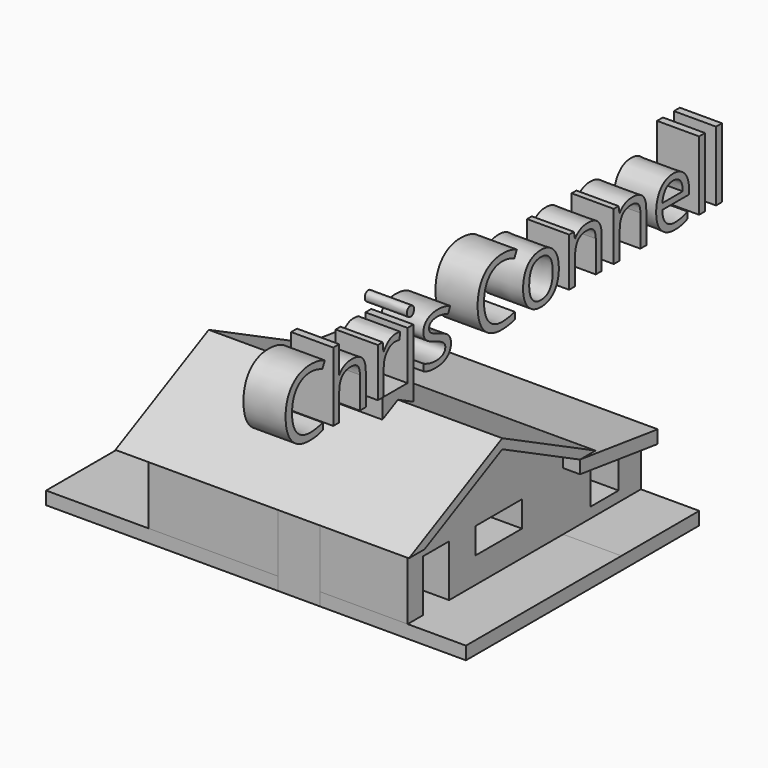
from build123d import *

# Parameters (mm, degrees)
F0_W           = 228.6
F0_H           = 101.6
F0_W_2         = 137.1599945068
F0_H_2         = 137.1599945068
F1_DEPTH       = 508
F0_W_3         = 76.2
F0_H_3         = 177.8
F2_DEPTH       = 530.86
F0_W_4         = 203.2000002861
F0_H_4         = 76.2000002861
F0_W_5         = 101.6
F3_DEPTH       = 736.6
F4_DEPTH       = 909.32
F0_TEXT_SIZE   = 356.014052199
F0_TEXT_SIZE_2 = 358.1658005713
F5_DEPTH       = 165.1
F6_DEPTH       = 25.4
F7_DEPTH       = 25.4
F8_DEPTH       = 25.4
F9_DEPTH       = 576.58
F9_DEPTH_BACK  = 574.04


# Not quite as in the source:
# - the program builds the solid bodies; features that only make, move or delete a surface that nothing else refers to are left out
# - Text() gives the source's letters only with a copy of the font that has no kerning and outlines rounded to 1/6400 em; it was checked with that copy


with BuildPart() as f1:
    # F0 (on Right) → F1 (new body, symmetric)
    with BuildSketch(Plane.YZ):
        Polygon((-381, 0), (0, 0), (0, 190.5), align=None)
        Polygon((0, 190.5), (0, 0), (381, 0), align=None)
        Polygon((381, 0), (0, 0), (-381, 0), (-381, -279.4), (-304.8, -279.4), (-304.8, -76.2), (-177.8, -76.2), (-177.8, -279.4), (381, -279.4), (381, -50.8), align=None)
        with Locations((65.0547002286, -127)):
            Rectangle(F0_W, F0_H, mode=Mode.SUBTRACT)
        Polygon((761.999634578, -101.072315), (381, -50.8), (381, -279.4), (761.999634578, -278.872315), align=None)
        with Locations((584.199634578, -170.049968493)):
            Rectangle(F0_W_2, F0_H_2, mode=Mode.SUBTRACT)
    extrude(amount=F1_DEPTH, both=True)


with BuildPart() as f2:
    # F0 (on Right) → F2 (new body)
    with BuildSketch(Plane.YZ):
        with Locations((-241.3, -190.5)):
            Rectangle(F0_W_3, F0_H_3)
    extrude(amount=-F2_DEPTH)


with BuildPart() as f2b:
    # F0 (on Right) → F2, piece 2 (new body)
    with BuildSketch(Plane.YZ):
        with Locations((65.0547002286, -127)):
            Rectangle(F0_W_4, F0_H_4)
    extrude(amount=-F2_DEPTH)

    # F6 (add): a face of the model
    f6_faces = [f2b.faces().sort_by_distance(p)[0] for p in [
        (-530.86, 65.0547002286, -127),
    ]]
    extrude(f6_faces, amount=F6_DEPTH)

    # F8 (add): a face of the model
    f8_faces = [f2b.faces().sort_by_distance(p)[0] for p in [
        (-556.26, 65.0547002286, -127),
    ]]
    extrude(f8_faces, amount=F8_DEPTH)


with BuildPart() as f2c:
    # F0 (on Right) → F2, piece 3 (new body)
    with BuildSketch(Plane.YZ):
        with Locations((584.199634578, -170.049968493)):
            Rectangle(F0_W_5, F0_H)
    extrude(amount=-F2_DEPTH)

    # F7 (add): a face of the model
    f7_faces = [f2c.faces().sort_by_distance(p)[0] for p in [
        (-530.86, 584.199634578, -170.049968493),
    ]]
    extrude(f7_faces, amount=F7_DEPTH)


with BuildPart() as f3:
    # F0 (on Right) → F3 (new body)
    with BuildSketch(Plane.YZ):
        Polygon((-304.8, -279.4), (-381, -279.4), (-381, -330.2), (381, -330.2), (381, -279.4), (-177.8, -279.4), (-203.2, -279.4), (-279.4, -279.4), align=None)
        Polygon((761.999634578, -278.872315), (381, -279.4), (381, -330.2), (762.069992578, -329.6722662771), align=None)
    extrude(amount=F3_DEPTH)


with BuildPart() as f4:
    # F0 (on Right) → F4 (new body)
    with BuildSketch(Plane.YZ):
        Polygon((-304.8, -279.4), (-381, -279.4), (-381, -330.2), (381, -330.2), (381, -279.4), (-177.8, -279.4), (-203.2, -279.4), (-279.4, -279.4), align=None)
        Polygon((761.999634578, -278.872315), (381, -279.4), (381, -330.2), (762.069992578, -329.6722662771), align=None)
    extrude(amount=-F4_DEPTH)


with BuildPart() as f5:
    # F0 (on Right) → F5 (new body)
    with BuildSketch(Plane.YZ):
        Polygon((381, 0), (0, 0), (-381, 0), (-381, -279.4), (-304.8, -279.4), (-304.8, -76.2), (-177.8, -76.2), (-177.8, -279.4), (381, -279.4), (381, -50.8), align=None)
        with Locations((65.0547002286, -127)):
            Rectangle(F0_W, F0_H, mode=Mode.SUBTRACT)
        Polygon((0, 190.5), (0, 0), (381, 0), align=None)
        Polygon((-381, 0), (0, 0), (0, 190.5), align=None)
        Polygon((-457.2, 0), (-381, 0), (0, 190.5), (0, 228.6), (-76.2, 190.5), align=None)
        Polygon((0, 190.5), (381, 0), (457.2, 0), (76.2, 190.5), (0, 228.6), align=None)
        Polygon((761.999634578, -50.272315), (381, 0), (381, -50.8), (761.999634578, -101.072315), align=None)
        Polygon((-304.8, -279.4), (-381, -279.4), (-381, -330.2), (381, -330.2), (381, -279.4), (-177.8, -279.4), (-203.2, -279.4), (-279.4, -279.4), align=None)
        Polygon((761.999634578, -101.072315), (381, -50.8), (381, -279.4), (761.999634578, -278.872315), align=None)
        with Locations((584.199634578, -170.049968493)):
            Rectangle(F0_W_2, F0_H_2, mode=Mode.SUBTRACT)
        Polygon((-76.2, 190.5), (0, 228.6), (76.2, 190.5), (76.2, 266.7), (75.864935357, 266.7), (46.9944208115, 266.7), (-69.4889268923, 266.7), (-76.2, 266.7), align=None)
        Polygon((761.999634578, -278.872315), (381, -279.4), (381, -330.2), (762.069992578, -329.6722662771), align=None)
        with Locations((-572.0806396451, 266.7)):
            Text('Chris Connel', F0_TEXT_SIZE, font='Open Sans', text_align=(TextAlign.LEFT, TextAlign.BOTTOM))
        with Locations((1527.7903691767, 265.150741172)):
            Text('l', F0_TEXT_SIZE_2, font='Open Sans', text_align=(TextAlign.LEFT, TextAlign.BOTTOM))
    extrude(amount=F5_DEPTH)


with BuildPart() as f9:
    # F0 (on Right) → F9 (new body, two sides)
    with BuildSketch(Plane.YZ) as f9_sk:
        Polygon((761.999634578, -50.272315), (381, 0), (381, -50.8), (761.999634578, -101.072315), align=None)
    extrude(amount=-F9_DEPTH)
    extrude(f9_sk.sketch, amount=F9_DEPTH_BACK)


with BuildPart() as f9b:
    # F0 (on Right) → F9, piece 2 (new body, two sides)
    with BuildSketch(Plane.YZ) as f9_2_sk:
        Polygon((0, 190.5), (381, 0), (457.2, 0), (76.2, 190.5), (0, 228.6), align=None)
        Polygon((-457.2, 0), (-381, 0), (0, 190.5), (0, 228.6), (-76.2, 190.5), align=None)
    extrude(amount=-F9_DEPTH)
    extrude(f9_2_sk.sketch, amount=F9_DEPTH_BACK)


solid = Compound([f1.part, f2.part, f2b.part, f2c.part, f3.part, f4.part, f5.part, f9.part, f9b.part])
